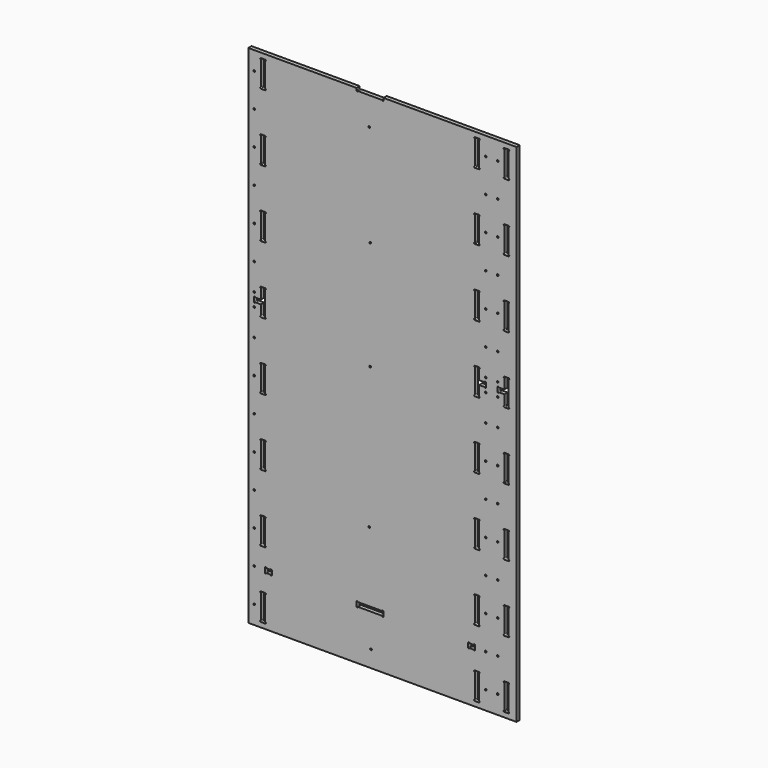
from build123d import *

# Parameters (mm, degrees)
F1_DEPTH = 18


# Not quite as in the source:
# - ends of sketch curves that miss each other by under 0.0002 mm in the source are joined


with BuildPart() as f1:
    # F0 (on Front) → F1 (new body)
    with BuildSketch(Plane.XZ):
        with BuildLine():
            Line((-600, 1063.948714), (-600, -1200))
            Line((-600, -1200), (599.500365, -1200))
            Line((599.500365, -1200), (599.501201, 1063.948476))
            Line((599.501201, 1063.948476), (4.500944, 1063.948707))
            Line((4.500944, 1063.948707), (4.50094, 1053.807502))
            ThreePointArc((4.50094, 1053.807502), (1.3610651837, 1050.5497977616), (-2.0190599785, 1053.5574880017))
            Line((-2.0190599785, 1053.5574880017), (-109.479176, 1053.557255))
            ThreePointArc((-109.479176, 1053.557255), (-112.8596545912, 1050.5399849452), (-115.9991760941, 1053.8072410001))
            Line((-115.9991760941, 1053.8072410001), (-115.999176, 1063.948687))
            Line((-115.999176, 1063.948687), (-600, 1063.948714))
        make_face()
        with BuildLine():
            ThreePointArc((-573.383933, -1114.274894), (-570.7322825706, -1115.3732435706), (-569.633933, -1118.024894))
            ThreePointArc((-569.633933, -1118.024894), (-570.7322825706, -1120.6765444294), (-573.383933, -1121.774894))
            ThreePointArc((-573.383933, -1121.774894), (-576.0355834294, -1120.6765444294), (-577.133933, -1118.024894))
            ThreePointArc((-577.133933, -1118.024894), (-576.0355834294, -1115.3732435706), (-573.383933, -1114.274894))
        make_face(mode=Mode.SUBTRACT)
        with BuildLine():
            ThreePointArc((-543.7502670069, -1064.0442210894), (-546.7588704515, -1060.6682126778), (-543.500265, -1057.5328310434))
            Line((-543.500265, -1057.5328310434), (-525.000247, -1057.532838))
            ThreePointArc((-525.000247, -1057.532838), (-521.7426305, -1060.6682591922), (-524.7502490411, -1064.0442274664))
            Line((-524.7502490411, -1064.0442274664), (-524.750289, -1172.021568))
            ThreePointArc((-524.750289, -1172.021568), (-521.7416865676, -1175.3975768203), (-525.000292, -1178.5329579566))
            Line((-525.000292, -1178.5329579566), (-543.50031, -1178.532951))
            ThreePointArc((-543.50031, -1178.532951), (-546.7579265191, -1175.3975293096), (-543.7503069648, -1172.021561457))
            Line((-543.7503069648, -1172.021561457), (-543.7502670069, -1064.0442210894))
        make_face(mode=Mode.SUBTRACT)
        with BuildLine():
            ThreePointArc((-573.383933, -964.274894), (-570.7322825706, -965.3732435706), (-569.633933, -968.024894))
            ThreePointArc((-569.633933, -968.024894), (-570.7322825706, -970.6765444294), (-573.383933, -971.774894))
            ThreePointArc((-573.383933, -971.774894), (-576.0355834294, -970.6765444294), (-577.133933, -968.024894))
            ThreePointArc((-577.133933, -968.024894), (-576.0355834294, -965.3732435706), (-573.383933, -964.274894))
        make_face(mode=Mode.SUBTRACT)
        with BuildLine():
            ThreePointArc((-525.7517729621, -958.780464), (-522.6163503118, -955.5228484425), (-519.2403833804, -958.5304690293))
            Line((-519.2403833804, -958.5304690293), (-501.263133, -958.530483))
            ThreePointArc((-501.263133, -958.530483), (-497.8871231819, -955.5218816059), (-494.7517430436, -958.780488))
            Line((-494.7517430436, -958.780488), (-494.751749, -977.284406))
            ThreePointArc((-494.751749, -977.284406), (-497.8871691944, -980.5420234617), (-501.2631383898, -977.534405953))
            Line((-501.2631383898, -977.534405953), (-519.240389, -977.534407))
            ThreePointArc((-519.240389, -977.534407), (-522.6163963244, -980.5430114898), (-525.7517789568, -977.284407))
            Line((-525.7517789568, -977.284407), (-525.7517729621, -958.780464))
        make_face(mode=Mode.SUBTRACT)
        with BuildLine():
            ThreePointArc((-573.383933, -814.274894), (-570.7322825706, -815.3732435706), (-569.633933, -818.024894))
            ThreePointArc((-569.633933, -818.024894), (-570.7322825706, -820.6765444294), (-573.383933, -821.774894))
            ThreePointArc((-573.383933, -821.774894), (-576.0355834294, -820.6765444294), (-577.133933, -818.024894))
            ThreePointArc((-577.133933, -818.024894), (-576.0355834294, -815.3732435706), (-573.383933, -814.274894))
        make_face(mode=Mode.SUBTRACT)
        with BuildLine():
            ThreePointArc((-525.000135, -757.5321180377), (-521.7425184809, -760.6675396904), (-524.7501380352, -764.043507543))
            Line((-524.7501380352, -764.043507543), (-524.750179, -872.020644))
            ThreePointArc((-524.750179, -872.020644), (-521.7415765477, -875.3966522839), (-525.000181, -878.5320329566))
            Line((-525.000181, -878.5320329566), (-543.500198, -878.532027))
            ThreePointArc((-543.500198, -878.532027), (-546.7578145191, -875.3966053096), (-543.7501949648, -872.020637457))
            Line((-543.7501949648, -872.020637457), (-543.750156, -764.043501))
            ThreePointArc((-543.750156, -764.043501), (-546.7587584324, -760.6674921797), (-543.500153, -757.5321110434))
            Line((-543.500153, -757.5321110434), (-525.000135, -757.5321180377))
        make_face(mode=Mode.SUBTRACT)
        with BuildLine():
            ThreePointArc((-573.383933, -664.274894), (-570.7322825706, -665.3732435706), (-569.633933, -668.024894))
            ThreePointArc((-569.633933, -668.024894), (-570.7322825706, -670.6765444294), (-573.383933, -671.774894))
            ThreePointArc((-573.383933, -671.774894), (-576.0355834294, -670.6765444294), (-577.133933, -668.024894))
            ThreePointArc((-577.133933, -668.024894), (-576.0355834294, -665.3732435706), (-573.383933, -664.274894))
        make_face(mode=Mode.SUBTRACT)
        with BuildLine():
            ThreePointArc((-54.784835, -1125.619), (-53.6864854294, -1122.9673495706), (-51.034835, -1121.869))
            ThreePointArc((-51.034835, -1121.869), (-48.3831845706, -1122.9673495706), (-47.284835, -1125.619))
            ThreePointArc((-47.284835, -1125.619), (-48.3831845706, -1128.2706504294), (-51.034835, -1129.369))
            ThreePointArc((-51.034835, -1129.369), (-53.6864854294, -1128.2706504294), (-54.784835, -1125.619))
        make_face(mode=Mode.SUBTRACT)
        with BuildLine():
            ThreePointArc((-109.7399839106, -977.5343350069), (-113.1159923222, -980.5429384515), (-116.2513739566, -977.284333))
            Line((-116.2513739566, -977.284333), (-116.251368, -958.78084))
            ThreePointArc((-116.251368, -958.78084), (-113.1159463096, -955.5232234809), (-109.739978457, -958.5308430352))
            Line((-109.739978457, -958.5308430352), (-1.762634, -958.530882))
            ThreePointArc((-1.762634, -958.530882), (1.6133748203, -955.5222795676), (4.7487559566, -958.780885))
            Line((4.7487559566, -958.780885), (4.74875, -977.284377))
            ThreePointArc((4.74875, -977.284377), (1.6133288078, -980.5419935), (-1.7626394664, -977.5343749589))
            Line((-1.7626394664, -977.5343749589), (-109.7399839106, -977.5343350069))
        make_face(mode=Mode.SUBTRACT)
        with BuildLine():
            ThreePointArc((-62.295835, -646.677873), (-61.1974854294, -644.0262225706), (-58.545835, -642.927873))
            ThreePointArc((-58.545835, -642.927873), (-55.8941845706, -644.0262225706), (-54.795835, -646.677873))
            ThreePointArc((-54.795835, -646.677873), (-55.8941845706, -649.3295234294), (-58.545835, -650.427873))
            ThreePointArc((-58.545835, -650.427873), (-61.1974854294, -649.3295234294), (-62.295835, -646.677873))
        make_face(mode=Mode.SUBTRACT)
        with BuildLine():
            ThreePointArc((-573.383933, -514.274894), (-570.7322825706, -515.3732435706), (-569.633933, -518.024894))
            ThreePointArc((-569.633933, -518.024894), (-570.7322825706, -520.6765444294), (-573.383933, -521.774894))
            ThreePointArc((-573.383933, -521.774894), (-576.0355834294, -520.6765444294), (-577.133933, -518.024894))
            ThreePointArc((-577.133933, -518.024894), (-576.0355834294, -515.3732435706), (-573.383933, -514.274894))
        make_face(mode=Mode.SUBTRACT)
        with BuildLine():
            ThreePointArc((-525.000025, -457.5316080377), (-521.7424085015, -460.6670291538), (-524.7500269645, -464.0429974605))
            Line((-524.7500269645, -464.0429974605), (-524.750068, -572.020134))
            ThreePointArc((-524.750068, -572.020134), (-521.7414655477, -575.3961422839), (-525.00007, -578.5315229566))
            Line((-525.00007, -578.5315229566), (-543.500087, -578.531516))
            ThreePointArc((-543.500087, -578.531516), (-546.7577034985, -575.3960948462), (-543.7500850355, -572.0201265395))
            Line((-543.7500850355, -572.0201265395), (-543.750045, -464.04299))
            ThreePointArc((-543.750045, -464.04299), (-546.7586474523, -460.6669817161), (-543.500043, -457.5316010434))
            Line((-543.500043, -457.5316010434), (-525.000025, -457.5316080377))
        make_face(mode=Mode.SUBTRACT)
        with BuildLine():
            ThreePointArc((-573.383933, -364.274894), (-570.7322825706, -365.3732435706), (-569.633933, -368.024894))
            ThreePointArc((-569.633933, -368.024894), (-570.7322825706, -370.6765444294), (-573.383933, -371.774894))
            ThreePointArc((-573.383933, -371.774894), (-576.0355834294, -370.6765444294), (-577.133933, -368.024894))
            ThreePointArc((-577.133933, -368.024894), (-576.0355834294, -365.3732435706), (-573.383933, -364.274894))
        make_face(mode=Mode.SUBTRACT)
        with BuildLine():
            ThreePointArc((-573.383933, -214.274894), (-570.7322825706, -215.3732435706), (-569.633933, -218.024894))
            ThreePointArc((-569.633933, -218.024894), (-570.7322825706, -220.6765444294), (-573.383933, -221.774894))
            ThreePointArc((-573.383933, -221.774894), (-576.0355834294, -220.6765444294), (-577.133933, -218.024894))
            ThreePointArc((-577.133933, -218.024894), (-576.0355834294, -215.3732435706), (-573.383933, -214.274894))
        make_face(mode=Mode.SUBTRACT)
        with BuildLine():
            ThreePointArc((-524.999914, -157.5310970377), (-521.7422974809, -160.6665186904), (-524.7499170352, -164.042486543))
            Line((-524.7499170352, -164.042486543), (-524.749957, -272.019623))
            ThreePointArc((-524.749957, -272.019623), (-521.7413545676, -275.3956318203), (-524.99996, -278.5310129566))
            Line((-524.99996, -278.5310129566), (-543.499977, -278.531006))
            ThreePointArc((-543.499977, -278.531006), (-546.7575935191, -275.3955843096), (-543.7499739648, -272.019616457))
            Line((-543.7499739648, -272.019616457), (-543.749934, -164.04248))
            ThreePointArc((-543.749934, -164.04248), (-546.7585364523, -160.6664717161), (-543.499932, -157.5310910434))
            Line((-543.499932, -157.5310910434), (-524.999914, -157.5310970377))
        make_face(mode=Mode.SUBTRACT)
        with BuildLine():
            ThreePointArc((-573.383933, -64.274894), (-570.7322825706, -65.3732435706), (-569.633933, -68.024894))
            ThreePointArc((-569.633933, -68.024894), (-570.7322825706, -70.6765444294), (-573.383933, -71.774894))
            ThreePointArc((-573.383933, -71.774894), (-576.0355834294, -70.6765444294), (-577.133933, -68.024894))
            ThreePointArc((-577.133933, -68.024894), (-576.0355834294, -65.3732435706), (-573.383933, -64.274894))
        make_face(mode=Mode.SUBTRACT)
        with BuildLine():
            ThreePointArc((-58.540835, -13.997), (-57.4424854294, -11.3453495706), (-54.790835, -10.247))
            ThreePointArc((-54.790835, -10.247), (-52.1391845706, -11.3453495706), (-51.040835, -13.997))
            ThreePointArc((-51.040835, -13.997), (-52.1391845706, -16.6486504294), (-54.790835, -17.747))
            ThreePointArc((-54.790835, -17.747), (-57.4424854294, -16.6486504294), (-58.540835, -13.997))
        make_face(mode=Mode.SUBTRACT)
        with BuildLine():
            ThreePointArc((413.2504909931, -1064.0491890894), (410.2418875485, -1060.6731806778), (413.500493, -1057.5377990434))
            Line((413.500493, -1057.5377990434), (432.000511, -1057.537806))
            ThreePointArc((432.000511, -1057.537806), (435.2581275, -1060.6732271922), (432.2505089589, -1064.0491954664))
            Line((432.2505089589, -1064.0491954664), (432.250469, -1172.026588))
            ThreePointArc((432.250469, -1172.026588), (435.2590714523, -1175.4025962839), (432.000467, -1178.5379769566))
            Line((432.000467, -1178.5379769566), (413.500449, -1178.53797))
            ThreePointArc((413.500449, -1178.53797), (410.2428325, -1175.4025488078), (413.2504510411, -1172.0265805336))
            Line((413.2504510411, -1172.0265805336), (413.2504909931, -1064.0491890894))
        make_face(mode=Mode.SUBTRACT)
        with BuildLine():
            ThreePointArc((389.7605140923, -977.5343449303), (386.3845067161, -980.5429474523), (383.2491260434, -977.284343))
            Line((383.2491260434, -977.284343), (383.249131, -958.781199))
            ThreePointArc((383.249131, -958.781199), (386.3845521922, -955.5235825), (389.7605204664, -958.5312010411))
            Line((389.7605204664, -958.5312010411), (407.737775, -958.531208))
            ThreePointArc((407.737775, -958.531208), (411.1137833222, -955.5226045485), (414.2491649566, -958.78121))
            Line((414.2491649566, -958.78121), (414.249159, -977.284354))
            ThreePointArc((414.249159, -977.284354), (411.1137378462, -980.5419704985), (407.7377695395, -977.5343520355))
            Line((407.7377695395, -977.5343520355), (389.7605140923, -977.5343449303))
        make_face(mode=Mode.SUBTRACT)
        with BuildLine():
            ThreePointArc((461.992664, -1114.274894), (464.6443144294, -1115.3732435706), (465.742664, -1118.024894))
            ThreePointArc((465.742664, -1118.024894), (464.6443144294, -1120.6765444294), (461.992664, -1121.774894))
            ThreePointArc((461.992664, -1121.774894), (459.3410135706, -1120.6765444294), (458.242664, -1118.024894))
            ThreePointArc((458.242664, -1118.024894), (459.3410135706, -1115.3732435706), (461.992664, -1114.274894))
        make_face(mode=Mode.SUBTRACT)
        with BuildLine():
            ThreePointArc((515.501328, -1114.274894), (518.1529784294, -1115.3732435706), (519.251328, -1118.024894))
            ThreePointArc((519.251328, -1118.024894), (518.1529784294, -1120.6765444294), (515.501328, -1121.774894))
            ThreePointArc((515.501328, -1121.774894), (512.8496775706, -1120.6765444294), (511.751328, -1118.024894))
            ThreePointArc((511.751328, -1118.024894), (512.8496775706, -1115.3732435706), (515.501328, -1114.274894))
        make_face(mode=Mode.SUBTRACT)
        with BuildLine():
            Line((545.250583, -1172.026629), (545.250623, -1064.049237))
            ThreePointArc((545.250623, -1064.049237), (542.2420205477, -1060.6732287161), (545.500625, -1057.5378480434))
            Line((545.500625, -1057.5378480434), (564.000643, -1057.537854))
            ThreePointArc((564.000643, -1057.537854), (567.2582595, -1060.6732751922), (564.2506409589, -1064.0492434664))
            Line((564.2506409589, -1064.0492434664), (564.250601, -1172.026636))
            ThreePointArc((564.250601, -1172.026636), (567.2592044515, -1175.4026443222), (564.000599, -1178.5380259566))
            Line((564.000599, -1178.5380259566), (545.500581, -1178.538019))
            ThreePointArc((545.500581, -1178.538019), (542.2429645, -1175.4025978078), (545.250583, -1172.026629))
        make_face(mode=Mode.SUBTRACT)
        with BuildLine():
            ThreePointArc((461.992664, -964.274894), (464.6443144294, -965.3732435706), (465.742664, -968.024894))
            ThreePointArc((465.742664, -968.024894), (464.6443144294, -970.6765444294), (461.992664, -971.774894))
            ThreePointArc((461.992664, -971.774894), (459.3410135706, -970.6765444294), (458.242664, -968.024894))
            ThreePointArc((458.242664, -968.024894), (459.3410135706, -965.3732435706), (461.992664, -964.274894))
        make_face(mode=Mode.SUBTRACT)
        with BuildLine():
            ThreePointArc((515.501328, -964.274894), (518.1529784294, -965.3732435706), (519.251328, -968.024894))
            ThreePointArc((519.251328, -968.024894), (518.1529784294, -970.6765444294), (515.501328, -971.774894))
            ThreePointArc((515.501328, -971.774894), (512.8496775706, -970.6765444294), (511.751328, -968.024894))
            ThreePointArc((511.751328, -968.024894), (512.8496775706, -965.3732435706), (515.501328, -964.274894))
        make_face(mode=Mode.SUBTRACT)
        with BuildLine():
            ThreePointArc((432.000622, -757.5278040377), (435.2582385, -760.6632251922), (432.2506199589, -764.0391934664))
            Line((432.2506199589, -764.0391934664), (432.25058, -872.016382))
            ThreePointArc((432.25058, -872.016382), (435.2591824324, -875.3923908204), (432.0005769998, -878.5277719566))
            Line((432.0005769998, -878.5277719566), (413.50056, -878.527765))
            ThreePointArc((413.50056, -878.527765), (410.2429434809, -875.3923433096), (413.2505630352, -872.016375457))
            Line((413.2505630352, -872.016375457), (413.250602, -764.039187))
            ThreePointArc((413.250602, -764.039187), (410.2419995477, -760.6631787161), (413.500604, -757.5277980434))
            Line((413.500604, -757.5277980434), (432.000622, -757.5278040377))
        make_face(mode=Mode.SUBTRACT)
        with BuildLine():
            ThreePointArc((461.992664, -814.274894), (464.6443144294, -815.3732435706), (465.742664, -818.024894))
            ThreePointArc((465.742664, -818.024894), (464.6443144294, -820.6765444294), (461.992664, -821.774894))
            ThreePointArc((461.992664, -821.774894), (459.3410135706, -820.6765444294), (458.242664, -818.024894))
            ThreePointArc((458.242664, -818.024894), (459.3410135706, -815.3732435706), (461.992664, -814.274894))
        make_face(mode=Mode.SUBTRACT)
        with BuildLine():
            ThreePointArc((515.501328, -814.274894), (518.1529784294, -815.3732435706), (519.251328, -818.024894))
            ThreePointArc((519.251328, -818.024894), (518.1529784294, -820.6765444294), (515.501328, -821.774894))
            ThreePointArc((515.501328, -821.774894), (512.8496775706, -820.6765444294), (511.751328, -818.024894))
            ThreePointArc((511.751328, -818.024894), (512.8496775706, -815.3732435706), (515.501328, -814.274894))
        make_face(mode=Mode.SUBTRACT)
        with BuildLine():
            ThreePointArc((545.500692, -878.5278129623), (542.2430754809, -875.3923913096), (545.2506950352, -872.016423457))
            Line((545.2506950352, -872.016423457), (545.250735, -764.039236))
            ThreePointArc((545.250735, -764.039236), (542.2421315485, -760.6632276778), (545.500737, -757.5278460434))
            Line((545.500737, -757.5278460434), (564.000755, -757.527853))
            ThreePointArc((564.000755, -757.527853), (567.2583715, -760.6632741922), (564.2507529589, -764.0392424664))
            Line((564.2507529589, -764.0392424664), (564.250713, -872.01643))
            ThreePointArc((564.250713, -872.01643), (567.2593154324, -875.3924388203), (564.00071, -878.5278199566))
            Line((564.00071, -878.5278199566), (545.500692, -878.5278129623))
        make_face(mode=Mode.SUBTRACT)
        with BuildLine():
            ThreePointArc((461.992664, -664.274894), (464.6443144294, -665.3732435706), (465.742664, -668.024894))
            ThreePointArc((465.742664, -668.024894), (464.6443144294, -670.6765444294), (461.992664, -671.774894))
            ThreePointArc((461.992664, -671.774894), (459.3410135706, -670.6765444294), (458.242664, -668.024894))
            ThreePointArc((458.242664, -668.024894), (459.3410135706, -665.3732435706), (461.992664, -664.274894))
        make_face(mode=Mode.SUBTRACT)
        with BuildLine():
            ThreePointArc((515.501328, -664.274894), (518.1529784294, -665.3732435706), (519.251328, -668.024894))
            ThreePointArc((519.251328, -668.024894), (518.1529784294, -670.6765444294), (515.501328, -671.774894))
            ThreePointArc((515.501328, -671.774894), (512.8496775706, -670.6765444294), (511.751328, -668.024894))
            ThreePointArc((511.751328, -668.024894), (512.8496775706, -665.3732435706), (515.501328, -664.274894))
        make_face(mode=Mode.SUBTRACT)
        with BuildLine():
            ThreePointArc((432.2506899303, -572.0158729077), (435.2592924523, -575.3918802839), (432.000688, -578.5272609566))
            Line((432.000688, -578.5272609566), (413.500671, -578.527254))
            ThreePointArc((413.500671, -578.527254), (410.2430545015, -575.3918328462), (413.2506729645, -572.0158645395))
            Line((413.2506729645, -572.0158645395), (413.250712, -464.038677))
            ThreePointArc((413.250712, -464.038677), (410.2421095676, -460.6626681797), (413.500715, -457.5272870434))
            Line((413.500715, -457.5272870434), (432.000733, -457.527294))
            ThreePointArc((432.000733, -457.527294), (435.2583495191, -460.6627156904), (432.2507299648, -464.038683543))
            Line((432.2507299648, -464.038683543), (432.2506899303, -572.0158729077))
        make_face(mode=Mode.SUBTRACT)
        with BuildLine():
            ThreePointArc((461.992664, -514.274894), (464.6443144294, -515.3732435706), (465.742664, -518.024894))
            ThreePointArc((465.742664, -518.024894), (464.6443144294, -520.6765444294), (461.992664, -521.774894))
            ThreePointArc((461.992664, -521.774894), (459.3410135706, -520.6765444294), (458.242664, -518.024894))
            ThreePointArc((458.242664, -518.024894), (459.3410135706, -515.3732435706), (461.992664, -514.274894))
        make_face(mode=Mode.SUBTRACT)
        with BuildLine():
            ThreePointArc((515.501328, -514.274894), (518.1529784294, -515.3732435706), (519.251328, -518.024894))
            ThreePointArc((519.251328, -518.024894), (518.1529784294, -520.6765444294), (515.501328, -521.774894))
            ThreePointArc((515.501328, -521.774894), (512.8496775706, -520.6765444294), (511.751328, -518.024894))
            ThreePointArc((511.751328, -518.024894), (512.8496775706, -515.3732435706), (515.501328, -514.274894))
        make_face(mode=Mode.SUBTRACT)
        with BuildLine():
            ThreePointArc((545.500802, -578.5275069623), (542.2431855015, -575.3920858462), (545.2508039645, -572.0161175395))
            Line((545.2508039645, -572.0161175395), (545.250844, -464.038726))
            ThreePointArc((545.250844, -464.038726), (542.2422415676, -460.6627171797), (545.500847, -457.5273360434))
            Line((545.500847, -457.5273360434), (564.000865, -457.527343))
            ThreePointArc((564.000865, -457.527343), (567.2584815191, -460.6627646904), (564.2508619648, -464.038732543))
            Line((564.2508619648, -464.038732543), (564.250822, -572.016125))
            ThreePointArc((564.250822, -572.016125), (567.2594244523, -575.3921332839), (564.00082, -578.5275139566))
            Line((564.00082, -578.5275139566), (545.500802, -578.5275069623))
        make_face(mode=Mode.SUBTRACT)
        with BuildLine():
            ThreePointArc((461.992664, -364.274894), (464.6443144294, -365.3732435706), (465.742664, -368.024894))
            ThreePointArc((465.742664, -368.024894), (464.6443144294, -370.6765444294), (461.992664, -371.774894))
            ThreePointArc((461.992664, -371.774894), (459.3410135706, -370.6765444294), (458.242664, -368.024894))
            ThreePointArc((458.242664, -368.024894), (459.3410135706, -365.3732435706), (461.992664, -364.274894))
        make_face(mode=Mode.SUBTRACT)
        with BuildLine():
            ThreePointArc((515.501328, -364.274894), (518.1529784294, -365.3732435706), (519.251328, -368.024894))
            ThreePointArc((519.251328, -368.024894), (518.1529784294, -370.6765444294), (515.501328, -371.774894))
            ThreePointArc((515.501328, -371.774894), (512.8496775706, -370.6765444294), (511.751328, -368.024894))
            ThreePointArc((511.751328, -368.024894), (512.8496775706, -365.3732435706), (515.501328, -364.274894))
        make_face(mode=Mode.SUBTRACT)
        with BuildLine():
            ThreePointArc((432.000843, -157.5267840377), (435.2584595, -160.6622051922), (432.2508409589, -164.0381734664))
            Line((432.2508409589, -164.0381734664), (432.250801, -272.015361))
            ThreePointArc((432.250801, -272.015361), (435.2594044515, -275.3913693222), (432.000799, -278.5267509566))
            Line((432.000799, -278.5267509566), (413.500782, -278.526744))
            ThreePointArc((413.500782, -278.526744), (410.2431655, -275.3913228078), (413.2507840411, -272.0153545336))
            Line((413.2507840411, -272.0153545336), (413.250823, -164.038167))
            ThreePointArc((413.250823, -164.038167), (410.2422195485, -160.6621586778), (413.500825, -157.5267770434))
            Line((413.500825, -157.5267770434), (432.000843, -157.5267840377))
        make_face(mode=Mode.SUBTRACT)
        with BuildLine():
            ThreePointArc((461.992664, -214.274894), (464.6443144294, -215.3732435706), (465.742664, -218.024894))
            ThreePointArc((465.742664, -218.024894), (464.6443144294, -220.6765444294), (461.992664, -221.774894))
            ThreePointArc((461.992664, -221.774894), (459.3410135706, -220.6765444294), (458.242664, -218.024894))
            ThreePointArc((458.242664, -218.024894), (459.3410135706, -215.3732435706), (461.992664, -214.274894))
        make_face(mode=Mode.SUBTRACT)
        with BuildLine():
            ThreePointArc((515.501328, -214.274894), (518.1529784294, -215.3732435706), (519.251328, -218.024894))
            ThreePointArc((519.251328, -218.024894), (518.1529784294, -220.6765444294), (515.501328, -221.774894))
            ThreePointArc((515.501328, -221.774894), (512.8496775706, -220.6765444294), (511.751328, -218.024894))
            ThreePointArc((511.751328, -218.024894), (512.8496775706, -215.3732435706), (515.501328, -214.274894))
        make_face(mode=Mode.SUBTRACT)
        with BuildLine():
            ThreePointArc((564.000975, -157.5268330377), (567.2585915, -160.6622541922), (564.2509729589, -164.0382224664))
            Line((564.2509729589, -164.0382224664), (564.250933, -272.015614))
            ThreePointArc((564.250933, -272.015614), (567.2595364515, -275.3916223222), (564.000931, -278.5270039566))
            Line((564.000931, -278.5270039566), (545.500913, -278.526997))
            ThreePointArc((545.500913, -278.526997), (542.2432965, -275.3915758078), (545.2509150411, -272.0156075336))
            Line((545.2509150411, -272.0156075336), (545.250955, -164.038216))
            ThreePointArc((545.250955, -164.038216), (542.2423515485, -160.6622076778), (545.500957, -157.5268260434))
            Line((545.500957, -157.5268260434), (564.000975, -157.5268330377))
        make_face(mode=Mode.SUBTRACT)
        with BuildLine():
            ThreePointArc((461.992664, -64.274894), (464.6443144294, -65.3732435706), (465.742664, -68.024894))
            ThreePointArc((465.742664, -68.024894), (464.6443144294, -70.6765444294), (461.992664, -71.774894))
            ThreePointArc((461.992664, -71.774894), (459.3410135706, -70.6765444294), (458.242664, -68.024894))
            ThreePointArc((458.242664, -68.024894), (459.3410135706, -65.3732435706), (461.992664, -64.274894))
        make_face(mode=Mode.SUBTRACT)
        with BuildLine():
            ThreePointArc((515.501328, -64.274894), (518.1529784294, -65.3732435706), (519.251328, -68.024894))
            ThreePointArc((519.251328, -68.024894), (518.1529784294, -70.6765444294), (515.501328, -71.774894))
            ThreePointArc((515.501328, -71.774894), (512.8496775706, -70.6765444294), (511.751328, -68.024894))
            ThreePointArc((511.751328, -68.024894), (512.8496775706, -65.3732435706), (515.501328, -64.274894))
        make_face(mode=Mode.SUBTRACT)
        with BuildLine():
            ThreePointArc((-573.383933, 55.725106), (-570.7322825706, 54.6267564294), (-569.633933, 51.975106))
            ThreePointArc((-569.633933, 51.975106), (-570.7322825706, 49.3234555706), (-573.383933, 48.225106))
            ThreePointArc((-573.383933, 48.225106), (-576.0355834294, 49.3234555706), (-577.133933, 51.975106))
            ThreePointArc((-577.133933, 51.975106), (-576.0355834294, 54.6267564294), (-573.383933, 55.725106))
        make_face(mode=Mode.SUBTRACT)
        with BuildLine():
            ThreePointArc((-573.383933, 115.725106), (-570.7322825706, 114.6267564294), (-569.633933, 111.975106))
            ThreePointArc((-569.633933, 111.975106), (-570.7322825706, 109.3234555706), (-573.383933, 108.225106))
            ThreePointArc((-573.383933, 108.225106), (-576.0355834294, 109.3234555706), (-577.133933, 111.975106))
            ThreePointArc((-577.133933, 111.975106), (-576.0355834294, 114.6267564294), (-573.383933, 115.725106))
        make_face(mode=Mode.SUBTRACT)
        with BuildLine():
            ThreePointArc((-524.999803, 142.4694129623), (-521.7421864809, 139.3339913096), (-524.7498060352, 135.958023457))
            Line((-524.7498060352, 135.958023457), (-524.749847, 27.980887))
            ThreePointArc((-524.749847, 27.980887), (-521.7412435485, 24.6048786778), (-524.999849, 21.4694970434))
            Line((-524.999849, 21.4694970434), (-543.499866, 21.469504))
            ThreePointArc((-543.499866, 21.469504), (-546.7574825, 24.6049251922), (-543.7498639589, 27.9808934664))
            Line((-543.7498639589, 27.9808934664), (-543.749847, 72.46956))
            Line((-543.749847, 72.46956), (-568.238488, 72.469401))
            ThreePointArc((-568.238488, 72.469401), (-571.6144758305, 69.4607757234), (-574.7498789601, 72.71936))
            Line((-574.7498789601, 72.71936), (-574.749872, 91.21938))
            ThreePointArc((-574.749872, 91.21938), (-571.6144508462, 94.4769964985), (-568.2384825395, 91.4693780355))
            Line((-568.2384825395, 91.4693780355), (-543.749841, 91.469369))
            Line((-543.749841, 91.469369), (-543.749825, 135.95803))
            ThreePointArc((-543.749825, 135.95803), (-546.7584284515, 139.3340383222), (-543.499823, 142.4694199566))
            Line((-543.499823, 142.4694199566), (-524.999803, 142.4694129623))
        make_face(mode=Mode.SUBTRACT)
        with BuildLine():
            ThreePointArc((-573.383933, 235.725106), (-570.7322825706, 234.6267564294), (-569.633933, 231.975106))
            ThreePointArc((-569.633933, 231.975106), (-570.7322825706, 229.3234555706), (-573.383933, 228.225106))
            ThreePointArc((-573.383933, 228.225106), (-576.0355834294, 229.3234555706), (-577.133933, 231.975106))
            ThreePointArc((-577.133933, 231.975106), (-576.0355834294, 234.6267564294), (-573.383933, 235.725106))
        make_face(mode=Mode.SUBTRACT)
        with BuildLine():
            ThreePointArc((-573.383933, 385.725106), (-570.7322825706, 384.6267564294), (-569.633933, 381.975106))
            ThreePointArc((-569.633933, 381.975106), (-570.7322825706, 379.3234555706), (-573.383933, 378.225106))
            ThreePointArc((-573.383933, 378.225106), (-576.0355834294, 379.3234555706), (-577.133933, 381.975106))
            ThreePointArc((-577.133933, 381.975106), (-576.0355834294, 384.6267564294), (-573.383933, 385.725106))
        make_face(mode=Mode.SUBTRACT)
        with BuildLine():
            ThreePointArc((-524.999693, 442.4697639623), (-521.7420765, 439.3343428078), (-524.7496950411, 435.9583745336))
            Line((-524.7496950411, 435.9583745336), (-524.749736, 327.981238))
            ThreePointArc((-524.749736, 327.981238), (-521.7411335676, 324.6052291797), (-524.999739, 321.4698480434))
            Line((-524.999739, 321.4698480434), (-543.499755, 321.469855))
            ThreePointArc((-543.499755, 321.469855), (-546.7573715, 324.6052761922), (-543.7497529589, 327.9812444664))
            Line((-543.7497529589, 327.9812444664), (-543.749713, 435.958381))
            ThreePointArc((-543.749713, 435.958381), (-546.7583164515, 439.3343893222), (-543.499711, 442.4697709566))
            Line((-543.499711, 442.4697709566), (-524.999693, 442.4697639623))
        make_face(mode=Mode.SUBTRACT)
        with BuildLine():
            ThreePointArc((-573.383933, 535.725106), (-570.7322825706, 534.6267564294), (-569.633933, 531.975106))
            ThreePointArc((-569.633933, 531.975106), (-570.7322825706, 529.3234555706), (-573.383933, 528.225106))
            ThreePointArc((-573.383933, 528.225106), (-576.0355834294, 529.3234555706), (-577.133933, 531.975106))
            ThreePointArc((-577.133933, 531.975106), (-576.0355834294, 534.6267564294), (-573.383933, 535.725106))
        make_face(mode=Mode.SUBTRACT)
        Polygon((-119.019569, 112.977778), (-136.576902, 112.977778), (-136.576902, 132.948445), (-119.019569, 132.948445), (-118.525193, 132.945041), (-118.033689, 132.91609), (-117.545989, 132.861984), (-117.063027, 132.783111), (-116.585737, 132.679864), (-116.115053, 132.552632), (-115.651908, 132.401807), (-115.197236, 132.227778), (-114.751969, 132.030937), (-114.317043, 131.811674), (-113.89339, 131.57038), (-113.481944, 131.307445), (-113.083639, 131.02326), (-112.699407, 130.718215), (-112.330184, 130.392702), (-111.976902, 130.047111), (-111.636463, 129.695604), (-111.315392, 129.328674), (-111.014055, 128.947213), (-110.732819, 128.552111), (-110.472052, 128.14426), (-110.232121, 127.724549), (-110.013393, 127.293869), (-109.816236, 126.853111), (-109.641015, 126.403166), (-109.4881, 125.944924), (-109.357857, 125.479275), (-109.250652, 125.007111), (-109.166854, 124.529322), (-109.106829, 124.046799), (-109.070945, 123.560432), (-109.059569, 123.071111), (-109.056599, 122.56955), (-109.079439, 122.070497), (-109.127708, 121.574896), (-109.201027, 121.083695), (-109.299019, 120.597837), (-109.421303, 120.118268), (-109.567502, 119.645933), (-109.737236, 119.181778), (-109.930126, 118.726748), (-110.145793, 118.281788), (-110.383859, 117.847844), (-110.643944, 117.425861), (-110.92567, 117.016784), (-111.228657, 116.621559), (-111.552528, 116.241131), (-111.896902, 115.876445), (-112.25703, 115.532319), (-112.632798, 115.208189), (-113.023285, 114.904427), (-113.427569, 114.621403), (-113.844728, 114.359488), (-114.27384, 114.119054), (-114.713983, 113.900471), (-115.164236, 113.704111), (-115.623676, 113.530345), (-116.091381, 113.379544), (-116.566431, 113.252078), (-117.047902, 113.14832), (-117.534874, 113.068639), (-118.026423, 113.013408), (-118.521629, 112.982997), align=None, mode=Mode.SUBTRACT)
        Polygon((-83.35778, 92.431213), (-83.771569, 92.428445), (-84.191435, 92.425041), (-84.610405, 92.432281), (-85.028287, 92.450088), (-85.444887, 92.478387), (-85.860012, 92.517102), (-86.273469, 92.566158), (-86.685067, 92.625477), (-87.094611, 92.694986), (-87.501908, 92.774608), (-87.906767, 92.864268), (-88.308995, 92.96389), (-88.708397, 93.073398), (-89.104782, 93.192716), (-89.497956, 93.32177), (-89.887727, 93.460482), (-90.273902, 93.608778), (-90.656288, 93.766582), (-91.034692, 93.933818), (-91.408921, 94.11041), (-91.778782, 94.296283), (-92.144083, 94.491361), (-92.504631, 94.695569), (-92.860232, 94.90883), (-93.210694, 95.13107), (-93.555824, 95.362211), (-93.895429, 95.60218), (-94.229316, 95.850899), (-94.557293, 96.108294), (-94.879166, 96.374288), (-95.194743, 96.648806), (-95.50383, 96.931772), (-95.806236, 97.223111), (-96.156096, 97.603393), (-96.495617, 97.991581), (-96.824711, 98.387442), (-97.143288, 98.790742), (-97.451259, 99.201246), (-97.748536, 99.618723), (-98.03503, 100.042936), (-98.310652, 100.473653), (-98.575313, 100.910639), (-98.828924, 101.353661), (-99.071397, 101.802485), (-99.302642, 102.256877), (-99.52257, 102.716603), (-99.731094, 103.181428), (-99.928123, 103.65112), (-100.113569, 104.125445), (-100.287343, 104.604167), (-100.449357, 105.087055), (-100.599521, 105.573873), (-100.737746, 106.064387), (-100.863944, 106.558365), (-100.978026, 107.055572), (-101.079903, 107.555773), (-101.169486, 108.058736), (-101.246686, 108.564227), (-101.311414, 109.07201), (-101.363582, 109.581854), (-101.4031, 110.093523), (-101.42988, 110.606784), (-101.443833, 111.121402), (-101.44487, 111.637145), (-101.432902, 112.153778), (-101.448973, 112.714899), (-101.450751, 113.275089), (-101.438334, 113.834088), (-101.411819, 114.391637), (-101.371304, 114.947478), (-101.316887, 115.50135), (-101.248665, 116.052995), (-101.166736, 116.602153), (-101.071197, 117.148565), (-100.962147, 117.691971), (-100.839683, 118.232113), (-100.703902, 118.768731), (-100.554903, 119.301566), (-100.392782, 119.830358), (-100.217639, 120.354849), (-100.029569, 120.874778), (-99.828671, 121.389887), (-99.615043, 121.899917), (-99.388782, 122.404607), (-99.149986, 122.9037), (-98.898752, 123.396935), (-98.635178, 123.884053), (-98.359362, 124.364796), (-98.071402, 124.838903), (-97.771395, 125.306116), (-97.459439, 125.766174), (-97.135631, 126.21882), (-96.800069, 126.663794), (-96.452851, 127.100835), (-96.094074, 127.529686), (-95.723836, 127.950087), (-95.342236, 128.361778), (-95.056487, 128.652452), (-94.763872, 128.934919), (-94.464585, 129.209099), (-94.158824, 129.474908), (-93.846783, 129.732267), (-93.528659, 129.981092), (-93.204648, 130.221304), (-92.874944, 130.45282), (-92.539744, 130.675558), (-92.199244, 130.889437), (-91.853639, 131.094377), (-91.503126, 131.290294), (-91.1479, 131.477107), (-90.788157, 131.654736), (-90.424092, 131.823098), (-90.055902, 131.982111), (-89.683782, 132.131695), (-89.307929, 132.271768), (-88.928537, 132.402248), (-88.545803, 132.523054), (-88.159923, 132.634104), (-87.771092, 132.735316), (-87.379506, 132.82661), (-86.985361, 132.907903), (-86.588852, 132.979114), (-86.190176, 133.040161), (-85.789529, 133.090964), (-85.387105, 133.131439), (-84.983102, 133.161507), (-84.577714, 133.181085), (-84.171138, 133.190091), (-83.763569, 133.188445), (-83.349321, 133.184771), (-82.936208, 133.170307), (-82.52443, 133.145137), (-82.114183, 133.109346), (-81.705668, 133.063017), (-81.299081, 133.006236), (-80.89462, 132.939086), (-80.492486, 132.861653), (-80.092874, 132.774021), (-79.695984, 132.676273), (-79.302014, 132.568496), (-78.911163, 132.450773), (-78.523627, 132.323188), (-78.139607, 132.185827), (-77.759299, 132.038773), (-77.382902, 131.882111), (-77.010615, 131.715926), (-76.642635, 131.540302), (-76.279161, 131.355323), (-75.920392, 131.161075), (-75.566524, 130.957641), (-75.217758, 130.745105), (-74.87429, 130.523554), (-74.536319, 130.29307), (-74.204043, 130.053738), (-73.877661, 129.805643), (-73.557371, 129.54887), (-73.243371, 129.283502), (-72.935859, 129.009624), (-72.635034, 128.727322), (-72.341093, 128.436678), (-72.054236, 128.137778), (-71.684056, 127.72825), (-71.325077, 127.310335), (-70.977391, 126.884286), (-70.64109, 126.450356), (-70.316265, 126.0088), (-70.003009, 125.55987), (-69.701413, 125.10382), (-69.411569, 124.640903), (-69.133569, 124.171373), (-68.867504, 123.695483), (-68.613466, 123.213487), (-68.371548, 122.725637), (-68.141841, 122.232188), (-67.924436, 121.733393), (-67.719426, 121.229505), (-67.526902, 120.720778), (-67.346957, 120.207465), (-67.179681, 119.689819), (-67.025167, 119.168094), (-66.883506, 118.642544), (-66.754791, 118.113421), (-66.639113, 117.580979), (-66.536564, 117.045472), (-66.447236, 116.507153), (-66.37122, 115.966275), (-66.308608, 115.423092), (-66.259492, 114.877858), (-66.223965, 114.330825), (-66.202117, 113.782247), (-66.19404, 113.232378), (-66.199827, 112.68147), (-66.219569, 112.129778), (-66.21114, 111.61495), (-66.21579, 111.101125), (-66.233429, 110.588539), (-66.263965, 110.077429), (-66.307305, 109.568032), (-66.363358, 109.060585), (-66.432032, 108.555324), (-66.513236, 108.052486), (-66.606876, 107.552309), (-66.712863, 107.055029), (-66.831104, 106.560882), (-66.961506, 106.070106), (-67.103979, 105.582938), (-67.258431, 105.099613), (-67.424769, 104.62037), (-67.602902, 104.145445), (-67.792738, 103.675074), (-67.994186, 103.209495), (-68.207153, 102.748944), (-68.431548, 102.293658), (-68.667279, 101.843874), (-68.914254, 101.399829), (-69.172381, 100.96176), (-69.441569, 100.529903), (-69.721725, 100.104495), (-70.012759, 99.685773), (-70.314578, 99.273975), (-70.62709, 98.869335), (-70.950203, 98.472093), (-71.283827, 98.082483), (-71.627868, 97.700744), (-71.982236, 97.327111), (-72.276142, 97.035898), (-72.576735, 96.75281), (-72.883827, 96.477926), (-73.19723, 96.211325), (-73.516757, 95.953085), (-73.842218, 95.703285), (-74.173426, 95.462004), (-74.510194, 95.22932), (-74.852332, 95.005311), (-75.199654, 94.790057), (-75.551971, 94.583636), (-75.909095, 94.386127), (-76.270838, 94.197608), (-76.637012, 94.018158), (-77.00743, 93.847855), (-77.381902, 93.686778), (-77.760242, 93.535006), (-78.142261, 93.392617), (-78.527771, 93.25969), (-78.916585, 93.136304), (-79.308513, 93.022537), (-79.703369, 92.918467), (-80.100964, 92.824174), (-80.501111, 92.739736), (-80.90362, 92.665232), (-81.308305, 92.60074), (-81.714977, 92.546338), (-82.123449, 92.502106), (-82.533532, 92.468122), (-82.945038, 92.444465), align=None, mode=Mode.SUBTRACT)
        Polygon((-39.112447, 92.431213), (-39.526236, 92.428445), (-39.946102, 92.425041), (-40.365072, 92.432281), (-40.782954, 92.450088), (-41.199553, 92.478387), (-41.614678, 92.517102), (-42.028136, 92.566158), (-42.439733, 92.625477), (-42.849277, 92.694986), (-43.256575, 92.774608), (-43.661434, 92.864268), (-44.063661, 92.96389), (-44.463064, 93.073398), (-44.859449, 93.192716), (-45.252623, 93.32177), (-45.642394, 93.460482), (-46.028569, 93.608778), (-46.410955, 93.766582), (-46.789359, 93.933818), (-47.163588, 94.11041), (-47.533449, 94.296283), (-47.89875, 94.491361), (-48.259297, 94.695569), (-48.614899, 94.90883), (-48.965361, 95.13107), (-49.310491, 95.362211), (-49.650096, 95.60218), (-49.983983, 95.850899), (-50.31196, 96.108294), (-50.633833, 96.374288), (-50.949409, 96.648806), (-51.258497, 96.931772), (-51.560902, 97.223111), (-51.910762, 97.603393), (-52.250284, 97.991581), (-52.579377, 98.387442), (-52.897954, 98.790742), (-53.205926, 99.201246), (-53.503203, 99.618723), (-53.789697, 100.042936), (-54.065319, 100.473653), (-54.32998, 100.910639), (-54.583591, 101.353661), (-54.826064, 101.802485), (-55.057308, 102.256877), (-55.277237, 102.716603), (-55.48576, 103.181428), (-55.682789, 103.65112), (-55.868236, 104.125445), (-56.04201, 104.604167), (-56.204023, 105.087055), (-56.354187, 105.573873), (-56.492413, 106.064387), (-56.618611, 106.558365), (-56.732693, 107.055572), (-56.834569, 107.555773), (-56.924152, 108.058736), (-57.001352, 108.564227), (-57.066081, 109.07201), (-57.118248, 109.581854), (-57.157767, 110.093523), (-57.184547, 110.606784), (-57.1985, 111.121402), (-57.199537, 111.637145), (-57.187569, 112.153778), (-57.20364, 112.714899), (-57.205418, 113.275089), (-57.193001, 113.834088), (-57.166486, 114.391637), (-57.125971, 114.947478), (-57.071553, 115.50135), (-57.003331, 116.052995), (-56.921402, 116.602153), (-56.825864, 117.148565), (-56.716814, 117.691971), (-56.594349, 118.232113), (-56.458569, 118.768731), (-56.30957, 119.301566), (-56.147449, 119.830358), (-55.972305, 120.354849), (-55.784236, 120.874778), (-55.583338, 121.389887), (-55.36971, 121.899917), (-55.143448, 122.404607), (-54.904652, 122.9037), (-54.653418, 123.396935), (-54.389845, 123.884053), (-54.114029, 124.364796), (-53.826069, 124.838903), (-53.526062, 125.306116), (-53.214105, 125.766174), (-52.890297, 126.21882), (-52.554736, 126.663794), (-52.207517, 127.100835), (-51.848741, 127.529686), (-51.478503, 127.950087), (-51.096902, 128.361778), (-50.811154, 128.652452), (-50.518538, 128.934919), (-50.219252, 129.209099), (-49.913491, 129.474908), (-49.60145, 129.732267), (-49.283326, 129.981092), (-48.959314, 130.221304), (-48.629611, 130.45282), (-48.294411, 130.675558), (-47.953911, 130.889437), (-47.608306, 131.094377), (-47.257793, 131.290294), (-46.902567, 131.477107), (-46.542823, 131.654736), (-46.178759, 131.823098), (-45.810569, 131.982111), (-45.438449, 132.131695), (-45.062596, 132.271768), (-44.683204, 132.402248), (-44.30047, 132.523054), (-43.914589, 132.634104), (-43.525758, 132.735316), (-43.134172, 132.82661), (-42.740027, 132.907903), (-42.343519, 132.979114), (-41.944843, 133.040161), (-41.544195, 133.090964), (-41.141772, 133.131439), (-40.737769, 133.161507), (-40.332381, 133.181085), (-39.925804, 133.190091), (-39.518236, 133.188445), (-39.103987, 133.184771), (-38.690875, 133.170307), (-38.279096, 133.145137), (-37.86885, 133.109346), (-37.460334, 133.063017), (-37.053747, 133.006236), (-36.649287, 132.939086), (-36.247152, 132.861653), (-35.847541, 132.774021), (-35.450651, 132.676273), (-35.056681, 132.568496), (-34.665829, 132.450773), (-34.278294, 132.323188), (-33.894273, 132.185827), (-33.513966, 132.038773), (-33.137569, 131.882111), (-32.765282, 131.715926), (-32.397302, 131.540302), (-32.033828, 131.355323), (-31.675058, 131.161075), (-31.321191, 130.957641), (-30.972424, 130.745105), (-30.628956, 130.523554), (-30.290986, 130.29307), (-29.95871, 130.053738), (-29.632328, 129.805643), (-29.312038, 129.54887), (-28.998038, 129.283502), (-28.690526, 129.009624), (-28.3897, 128.727322), (-28.09576, 128.436678), (-27.808902, 128.137778), (-27.438722, 127.72825), (-27.079743, 127.310335), (-26.732057, 126.884286), (-26.395756, 126.450356), (-26.070932, 126.0088), (-25.757676, 125.55987), (-25.45608, 125.10382), (-25.166236, 124.640903), (-24.888235, 124.171373), (-24.62217, 123.695483), (-24.368133, 123.213487), (-24.126215, 122.725637), (-23.896507, 122.232188), (-23.679103, 121.733393), (-23.474093, 121.229505), (-23.281569, 120.720778), (-23.101623, 120.207465), (-22.934348, 119.689819), (-22.779834, 119.168094), (-22.638173, 118.642544), (-22.509458, 118.113421), (-22.39378, 117.580979), (-22.291231, 117.045472), (-22.201902, 116.507153), (-22.125886, 115.966275), (-22.063275, 115.423092), (-22.014159, 114.877858), (-21.978631, 114.330825), (-21.956783, 113.782247), (-21.948707, 113.232378), (-21.954494, 112.68147), (-21.974236, 112.129778), (-21.965806, 111.61495), (-21.970457, 111.101125), (-21.988096, 110.588539), (-22.018631, 110.077429), (-22.061972, 109.568032), (-22.118025, 109.060585), (-22.186699, 108.555324), (-22.267902, 108.052486), (-22.361543, 107.552309), (-22.46753, 107.055029), (-22.58577, 106.560882), (-22.716173, 106.070106), (-22.858646, 105.582938), (-23.013098, 105.099613), (-23.179436, 104.62037), (-23.357569, 104.145445), (-23.547405, 103.675074), (-23.748853, 103.209495), (-23.96182, 102.748944), (-24.186215, 102.293658), (-24.421946, 101.843874), (-24.66892, 101.399829), (-24.927048, 100.96176), (-25.196236, 100.529903), (-25.476392, 100.104495), (-25.767426, 99.685773), (-26.069244, 99.273975), (-26.381756, 98.869335), (-26.70487, 98.472093), (-27.038493, 98.082483), (-27.382535, 97.700744), (-27.736902, 97.327111), (-28.030808, 97.035898), (-28.331402, 96.75281), (-28.638494, 96.477926), (-28.951897, 96.211325), (-29.271423, 95.953085), (-29.596885, 95.703285), (-29.928093, 95.462004), (-30.264861, 95.22932), (-30.606999, 95.005311), (-30.954321, 94.790057), (-31.306638, 94.583636), (-31.663762, 94.386127), (-32.025505, 94.197608), (-32.391679, 94.018158), (-32.762096, 93.847855), (-33.136569, 93.686778), (-33.514909, 93.535006), (-33.896928, 93.392617), (-34.282438, 93.25969), (-34.671251, 93.136304), (-35.06318, 93.022537), (-35.458036, 92.918467), (-35.855631, 92.824174), (-36.255777, 92.739736), (-36.658287, 92.665232), (-37.062972, 92.60074), (-37.469644, 92.546338), (-37.878116, 92.502106), (-38.288199, 92.468122), (-38.699705, 92.444465), align=None, mode=Mode.SUBTRACT)
        with BuildLine():
            ThreePointArc((-58.540835, 474.216), (-57.4424854294, 476.8676504294), (-54.790835, 477.966))
            ThreePointArc((-54.790835, 477.966), (-52.1391845706, 476.8676504294), (-51.040835, 474.216))
            ThreePointArc((-51.040835, 474.216), (-52.1391845706, 471.5643495706), (-54.790835, 470.466))
            ThreePointArc((-54.790835, 470.466), (-57.4424854294, 471.5643495706), (-58.540835, 474.216))
        make_face(mode=Mode.SUBTRACT)
        with BuildLine():
            ThreePointArc((-573.383933, 685.725106), (-570.7322825706, 684.6267564294), (-569.633933, 681.975106))
            ThreePointArc((-569.633933, 681.975106), (-570.7322825706, 679.3234555706), (-573.383933, 678.225106))
            ThreePointArc((-573.383933, 678.225106), (-576.0355834294, 679.3234555706), (-577.133933, 681.975106))
            ThreePointArc((-577.133933, 681.975106), (-576.0355834294, 684.6267564294), (-573.383933, 685.725106))
        make_face(mode=Mode.SUBTRACT)
        with BuildLine():
            ThreePointArc((-524.7496259931, 627.9817480894), (-521.7410225485, 624.6057396778), (-524.999628, 621.4703580434))
            Line((-524.999628, 621.4703580434), (-543.499645, 621.470365))
            ThreePointArc((-543.499645, 621.470365), (-546.7572615191, 624.6057866904), (-543.7496419648, 627.981754543))
            Line((-543.7496419648, 627.981754543), (-543.749603, 735.958891))
            ThreePointArc((-543.749603, 735.958891), (-546.7582054324, 739.3348998203), (-543.4996, 742.4702809566))
            Line((-543.4996, 742.4702809566), (-524.999582, 742.470274))
            ThreePointArc((-524.999582, 742.470274), (-521.7419654809, 739.3348523096), (-524.7495850352, 735.958884457))
            Line((-524.7495850352, 735.958884457), (-524.7496259931, 627.9817480894))
        make_face(mode=Mode.SUBTRACT)
        with BuildLine():
            ThreePointArc((-573.383933, 835.725106), (-570.7322825706, 834.6267564294), (-569.633933, 831.975106))
            ThreePointArc((-569.633933, 831.975106), (-570.7322825706, 829.3234555706), (-573.383933, 828.225106))
            ThreePointArc((-573.383933, 828.225106), (-576.0355834294, 829.3234555706), (-577.133933, 831.975106))
            ThreePointArc((-577.133933, 831.975106), (-576.0355834294, 834.6267564294), (-573.383933, 835.725106))
        make_face(mode=Mode.SUBTRACT)
        with BuildLine():
            ThreePointArc((-573.383933, 985.725106), (-570.7322825706, 984.6267564294), (-569.633933, 981.975106))
            ThreePointArc((-569.633933, 981.975106), (-570.7322825706, 979.3234555706), (-573.383933, 978.225106))
            ThreePointArc((-573.383933, 978.225106), (-576.0355834294, 979.3234555706), (-577.133933, 981.975106))
            ThreePointArc((-577.133933, 981.975106), (-576.0355834294, 984.6267564294), (-573.383933, 985.725106))
        make_face(mode=Mode.SUBTRACT)
        with BuildLine():
            ThreePointArc((-524.7495149931, 927.9822580894), (-521.7409115485, 924.6062496778), (-524.999517, 921.4708680434))
            Line((-524.999517, 921.4708680434), (-543.499534, 921.470875))
            ThreePointArc((-543.499534, 921.470875), (-546.7571505, 924.6062961922), (-543.7495319589, 927.9822644664))
            Line((-543.7495319589, 927.9822644664), (-543.749492, 1035.959401))
            ThreePointArc((-543.749492, 1035.959401), (-546.7580954515, 1039.3354093222), (-543.49949, 1042.4707909566))
            Line((-543.49949, 1042.4707909566), (-524.999472, 1042.470784))
            ThreePointArc((-524.999472, 1042.470784), (-521.7418555, 1039.3353628078), (-524.7494740411, 1035.9593945336))
            Line((-524.7494740411, 1035.9593945336), (-524.7495149931, 927.9822580894))
        make_face(mode=Mode.SUBTRACT)
        with BuildLine():
            ThreePointArc((-62.295835, 928.629), (-61.1974854294, 931.2806504294), (-58.545835, 932.379))
            ThreePointArc((-58.545835, 932.379), (-55.8941845706, 931.2806504294), (-54.795835, 928.629))
            ThreePointArc((-54.795835, 928.629), (-55.8941845706, 925.9773495706), (-58.545835, 924.879))
            ThreePointArc((-58.545835, 924.879), (-61.1974854294, 925.9773495706), (-62.295835, 928.629))
        make_face(mode=Mode.SUBTRACT)
        with BuildLine():
            ThreePointArc((432.250912001, 27.9788200131), (435.2595144324, 24.6028111797), (432.000909, 21.4674300434))
            Line((432.000909, 21.4674300434), (413.500892, 21.467437))
            ThreePointArc((413.500892, 21.467437), (410.2432754809, 24.6028586904), (413.2508950352, 27.978826543))
            Line((413.2508950352, 27.978826543), (413.250933, 135.956014))
            ThreePointArc((413.250933, 135.956014), (410.2423305676, 139.3320228203), (413.500936, 142.4674039566))
            Line((413.500936, 142.4674039566), (432.000954, 142.467397))
            ThreePointArc((432.000954, 142.467397), (435.2585705, 139.3319758078), (432.2509519589, 135.9560075336))
            Line((432.2509519589, 135.9560075336), (432.250936, 91.46753))
            Line((432.250936, 91.46753), (456.739578, 91.467353))
            ThreePointArc((456.739578, 91.467353), (460.1156068484, 94.4759325866), (463.2509659529, 91.217306))
            Line((463.2509659529, 91.217306), (463.250959, 72.717291))
            ThreePointArc((463.250959, 72.717291), (460.1155378078, 69.4596745), (456.7395695336, 72.4672930411))
            Line((456.7395695336, 72.4672930411), (432.250928, 72.467302))
            Line((432.250928, 72.467302), (432.250912001, 27.9788200131))
        make_face(mode=Mode.SUBTRACT)
        with BuildLine():
            ThreePointArc((461.992664, 55.725106), (464.6443144294, 54.6267564294), (465.742664, 51.975106))
            ThreePointArc((465.742664, 51.975106), (464.6443144294, 49.3234555706), (461.992664, 48.225106))
            ThreePointArc((461.992664, 48.225106), (459.3410135706, 49.3234555706), (458.242664, 51.975106))
            ThreePointArc((458.242664, 51.975106), (459.3410135706, 54.6267564294), (461.992664, 55.725106))
        make_face(mode=Mode.SUBTRACT)
        with BuildLine():
            ThreePointArc((515.501328, 55.725106), (518.1529784294, 54.6267564294), (519.251328, 51.975106))
            ThreePointArc((519.251328, 51.975106), (518.1529784294, 49.3234555706), (515.501328, 48.225106))
            ThreePointArc((515.501328, 48.225106), (512.8496775706, 49.3234555706), (511.751328, 51.975106))
            ThreePointArc((511.751328, 51.975106), (512.8496775706, 54.6267564294), (515.501328, 55.725106))
        make_face(mode=Mode.SUBTRACT)
        with BuildLine():
            ThreePointArc((461.992664, 115.725106), (464.6443144294, 114.6267564294), (465.742664, 111.975106))
            ThreePointArc((465.742664, 111.975106), (464.6443144294, 109.3234555706), (461.992664, 108.225106))
            ThreePointArc((461.992664, 108.225106), (459.3410135706, 109.3234555706), (458.242664, 111.975106))
            ThreePointArc((458.242664, 111.975106), (459.3410135706, 114.6267564294), (461.992664, 115.725106))
        make_face(mode=Mode.SUBTRACT)
        with BuildLine():
            ThreePointArc((515.501328, 115.725106), (518.1529784294, 114.6267564294), (519.251328, 111.975106))
            ThreePointArc((519.251328, 111.975106), (518.1529784294, 109.3234555706), (515.501328, 108.225106))
            ThreePointArc((515.501328, 108.225106), (512.8496775706, 109.3234555706), (511.751328, 111.975106))
            ThreePointArc((511.751328, 111.975106), (512.8496775706, 114.6267564294), (515.501328, 115.725106))
        make_face(mode=Mode.SUBTRACT)
        with BuildLine():
            ThreePointArc((545.501024, 21.4673880377), (542.2434074809, 24.6028096904), (545.2510270352, 27.978777543))
            Line((545.2510270352, 27.978777543), (545.251043, 72.46747))
            Line((545.251043, 72.46747), (520.762402, 72.467311))
            ThreePointArc((520.762402, 72.467311), (517.3864141695, 69.4586857234), (514.2510110399, 72.71727))
            Line((514.2510110399, 72.71727), (514.251018, 91.21729))
            ThreePointArc((514.251018, 91.21729), (517.3864391922, 94.4749065), (520.7624074664, 91.4672879589))
            Line((520.7624074664, 91.4672879589), (545.251049, 91.467279))
            Line((545.251049, 91.467279), (545.251065, 135.955966))
            ThreePointArc((545.251065, 135.955966), (542.2424625676, 139.3319748204), (545.5010680002, 142.4673559566))
            Line((545.5010680002, 142.4673559566), (564.001087, 142.467349))
            ThreePointArc((564.001087, 142.467349), (567.2587035191, 139.3319273096), (564.2510839648, 135.955959457))
            Line((564.2510839648, 135.955959457), (564.251044, 27.978771))
            ThreePointArc((564.251044, 27.978771), (567.2596464324, 24.6027621797), (564.001041, 21.4673810434))
            Line((564.001041, 21.4673810434), (545.501024, 21.4673880377))
        make_face(mode=Mode.SUBTRACT)
        with BuildLine():
            ThreePointArc((461.992664, 235.725106), (464.6443144294, 234.6267564294), (465.742664, 231.975106))
            ThreePointArc((465.742664, 231.975106), (464.6443144294, 229.3234555706), (461.992664, 228.225106))
            ThreePointArc((461.992664, 228.225106), (459.3410135706, 229.3234555706), (458.242664, 231.975106))
            ThreePointArc((458.242664, 231.975106), (459.3410135706, 234.6267564294), (461.992664, 235.725106))
        make_face(mode=Mode.SUBTRACT)
        with BuildLine():
            ThreePointArc((515.501328, 235.725106), (518.1529784294, 234.6267564294), (519.251328, 231.975106))
            ThreePointArc((519.251328, 231.975106), (518.1529784294, 229.3234555706), (515.501328, 228.225106))
            ThreePointArc((515.501328, 228.225106), (512.8496775706, 229.3234555706), (511.751328, 231.975106))
            ThreePointArc((511.751328, 231.975106), (512.8496775706, 234.6267564294), (515.501328, 235.725106))
        make_face(mode=Mode.SUBTRACT)
        with BuildLine():
            ThreePointArc((432.2510220069, 327.9855000894), (435.2596254515, 324.6094916778), (432.00102, 321.4741100434))
            Line((432.00102, 321.4741100434), (413.501003, 321.474117))
            ThreePointArc((413.501003, 321.474117), (410.2433865, 324.6095381922), (413.2510050411, 327.9855064664))
            Line((413.2510050411, 327.9855064664), (413.251044, 435.962694))
            ThreePointArc((413.251044, 435.962694), (410.2424405485, 439.3387023222), (413.501046, 442.4740839566))
            Line((413.501046, 442.4740839566), (432.001064, 442.474077))
            ThreePointArc((432.001064, 442.474077), (435.2586805, 439.3386558078), (432.2510619589, 435.9626875336))
            Line((432.2510619589, 435.9626875336), (432.2510220069, 327.9855000894))
        make_face(mode=Mode.SUBTRACT)
        with BuildLine():
            ThreePointArc((461.992664, 385.725106), (464.6443144294, 384.6267564294), (465.742664, 381.975106))
            ThreePointArc((465.742664, 381.975106), (464.6443144294, 379.3234555706), (461.992664, 378.225106))
            ThreePointArc((461.992664, 378.225106), (459.3410135706, 379.3234555706), (458.242664, 381.975106))
            ThreePointArc((458.242664, 381.975106), (459.3410135706, 384.6267564294), (461.992664, 385.725106))
        make_face(mode=Mode.SUBTRACT)
        with BuildLine():
            ThreePointArc((515.501328, 385.725106), (518.1529784294, 384.6267564294), (519.251328, 381.975106))
            ThreePointArc((519.251328, 381.975106), (518.1529784294, 379.3234555706), (515.501328, 378.225106))
            ThreePointArc((515.501328, 378.225106), (512.8496775706, 379.3234555706), (511.751328, 381.975106))
            ThreePointArc((511.751328, 381.975106), (512.8496775706, 384.6267564294), (515.501328, 385.725106))
        make_face(mode=Mode.SUBTRACT)
        with BuildLine():
            ThreePointArc((545.501134, 321.4738640377), (542.2435175, 324.6092851922), (545.2511360411, 327.9852534664))
            Line((545.2511360411, 327.9852534664), (545.251176, 435.962646))
            ThreePointArc((545.251176, 435.962646), (542.2425735477, 439.3386542839), (545.501178, 442.4740349566))
            Line((545.501178, 442.4740349566), (564.001196, 442.474028))
            ThreePointArc((564.001196, 442.474028), (567.2588124985, 439.3386068462), (564.2511940355, 435.9626385395))
            Line((564.2511940355, 435.9626385395), (564.251154, 327.985247))
            ThreePointArc((564.251154, 327.985247), (567.2597574515, 324.6092386778), (564.001152, 321.4738570434))
            Line((564.001152, 321.4738570434), (545.501134, 321.4738640377))
        make_face(mode=Mode.SUBTRACT)
        with BuildLine():
            ThreePointArc((461.992664, 535.725106), (464.6443144294, 534.6267564294), (465.742664, 531.975106))
            ThreePointArc((465.742664, 531.975106), (464.6443144294, 529.3234555706), (461.992664, 528.225106))
            ThreePointArc((461.992664, 528.225106), (459.3410135706, 529.3234555706), (458.242664, 531.975106))
            ThreePointArc((458.242664, 531.975106), (459.3410135706, 534.6267564294), (461.992664, 535.725106))
        make_face(mode=Mode.SUBTRACT)
        with BuildLine():
            ThreePointArc((515.501328, 535.725106), (518.1529784294, 534.6267564294), (519.251328, 531.975106))
            ThreePointArc((519.251328, 531.975106), (518.1529784294, 529.3234555706), (515.501328, 528.225106))
            ThreePointArc((515.501328, 528.225106), (512.8496775706, 529.3234555706), (511.751328, 531.975106))
            ThreePointArc((511.751328, 531.975106), (512.8496775706, 534.6267564294), (515.501328, 535.725106))
        make_face(mode=Mode.SUBTRACT)
        with BuildLine():
            ThreePointArc((432.251133001, 627.9860100131), (435.2597354324, 624.6100011797), (432.00113, 621.4746200434))
            Line((432.00113, 621.4746200434), (413.501113, 621.474627))
            ThreePointArc((413.501113, 621.474627), (410.2434964809, 624.6100486904), (413.2511160352, 627.986016543))
            Line((413.2511160352, 627.986016543), (413.251155, 735.963204))
            ThreePointArc((413.251155, 735.963204), (410.2425515485, 739.3392123222), (413.501157, 742.4745939566))
            Line((413.501157, 742.4745939566), (432.001175, 742.474587))
            ThreePointArc((432.001175, 742.474587), (435.2587915, 739.3391658078), (432.2511729589, 735.9631975336))
            Line((432.2511729589, 735.9631975336), (432.251133001, 627.9860100131))
        make_face(mode=Mode.SUBTRACT)
        with BuildLine():
            ThreePointArc((461.992664, 685.725106), (464.6443144294, 684.6267564294), (465.742664, 681.975106))
            ThreePointArc((465.742664, 681.975106), (464.6443144294, 679.3234555706), (461.992664, 678.225106))
            ThreePointArc((461.992664, 678.225106), (459.3410135706, 679.3234555706), (458.242664, 681.975106))
            ThreePointArc((458.242664, 681.975106), (459.3410135706, 684.6267564294), (461.992664, 685.725106))
        make_face(mode=Mode.SUBTRACT)
        with BuildLine():
            ThreePointArc((515.501328, 685.725106), (518.1529784294, 684.6267564294), (519.251328, 681.975106))
            ThreePointArc((519.251328, 681.975106), (518.1529784294, 679.3234555706), (515.501328, 678.225106))
            ThreePointArc((515.501328, 678.225106), (512.8496775706, 679.3234555706), (511.751328, 681.975106))
            ThreePointArc((511.751328, 681.975106), (512.8496775706, 684.6267564294), (515.501328, 685.725106))
        make_face(mode=Mode.SUBTRACT)
        with BuildLine():
            ThreePointArc((545.501244, 621.4743740377), (542.2436274809, 624.6097956904), (545.2512470352, 627.985763543))
            Line((545.2512470352, 627.985763543), (545.251287, 735.963156))
            ThreePointArc((545.251287, 735.963156), (542.2426845477, 739.3391642839), (545.501289, 742.4745449566))
            Line((545.501289, 742.4745449566), (564.001307, 742.474539))
            ThreePointArc((564.001307, 742.474539), (567.2589235, 739.3391178078), (564.2513049589, 735.9631495336))
            Line((564.2513049589, 735.9631495336), (564.251265, 627.985757))
            ThreePointArc((564.251265, 627.985757), (567.2598674324, 624.6097481797), (564.001262, 621.4743670434))
            Line((564.001262, 621.4743670434), (545.501244, 621.4743740377))
        make_face(mode=Mode.SUBTRACT)
        with BuildLine():
            ThreePointArc((461.992664, 835.725106), (464.6443144294, 834.6267564294), (465.742664, 831.975106))
            ThreePointArc((465.742664, 831.975106), (464.6443144294, 829.3234555706), (461.992664, 828.225106))
            ThreePointArc((461.992664, 828.225106), (459.3410135706, 829.3234555706), (458.242664, 831.975106))
            ThreePointArc((458.242664, 831.975106), (459.3410135706, 834.6267564294), (461.992664, 835.725106))
        make_face(mode=Mode.SUBTRACT)
        with BuildLine():
            ThreePointArc((515.501328, 835.725106), (518.1529784294, 834.6267564294), (519.251328, 831.975106))
            ThreePointArc((519.251328, 831.975106), (518.1529784294, 829.3234555706), (515.501328, 828.225106))
            ThreePointArc((515.501328, 828.225106), (512.8496775706, 829.3234555706), (511.751328, 831.975106))
            ThreePointArc((511.751328, 831.975106), (512.8496775706, 834.6267564294), (515.501328, 835.725106))
        make_face(mode=Mode.SUBTRACT)
        with BuildLine():
            ThreePointArc((432.2512429303, 927.9859070923), (435.2598454523, 924.6098997161), (432.001241, 921.4745190434))
            Line((432.001241, 921.4745190434), (413.501223, 921.474525))
            ThreePointArc((413.501223, 921.474525), (410.2436065, 924.6099461922), (413.2512250411, 927.9859144664))
            Line((413.2512250411, 927.9859144664), (413.251265, 1035.963307))
            ThreePointArc((413.251265, 1035.963307), (410.2426625676, 1039.3393158203), (413.501268, 1042.4746969566))
            Line((413.501268, 1042.4746969566), (432.001287, 1042.47469))
            ThreePointArc((432.001287, 1042.47469), (435.2589035191, 1039.3392683096), (432.2512839648, 1035.963300457))
            Line((432.2512839648, 1035.963300457), (432.2512429303, 927.9859070923))
        make_face(mode=Mode.SUBTRACT)
        with BuildLine():
            ThreePointArc((461.992664, 985.725106), (464.6443144294, 984.6267564294), (465.742664, 981.975106))
            ThreePointArc((465.742664, 981.975106), (464.6443144294, 979.3234555706), (461.992664, 978.225106))
            ThreePointArc((461.992664, 978.225106), (459.3410135706, 979.3234555706), (458.242664, 981.975106))
            ThreePointArc((458.242664, 981.975106), (459.3410135706, 984.6267564294), (461.992664, 985.725106))
        make_face(mode=Mode.SUBTRACT)
        with BuildLine():
            ThreePointArc((515.501328, 985.725106), (518.1529784294, 984.6267564294), (519.251328, 981.975106))
            ThreePointArc((519.251328, 981.975106), (518.1529784294, 979.3234555706), (515.501328, 978.225106))
            ThreePointArc((515.501328, 978.225106), (512.8496775706, 979.3234555706), (511.751328, 981.975106))
            ThreePointArc((511.751328, 981.975106), (512.8496775706, 984.6267564294), (515.501328, 985.725106))
        make_face(mode=Mode.SUBTRACT)
        with BuildLine():
            ThreePointArc((545.501356, 921.4746810377), (542.2437395, 924.6101021922), (545.2513580411, 927.9860704664))
            Line((545.2513580411, 927.9860704664), (545.251398, 1035.963258))
            ThreePointArc((545.251398, 1035.963258), (542.2427955676, 1039.3392668203), (545.501401, 1042.4746479566))
            Line((545.501401, 1042.4746479566), (564.001419, 1042.474641))
            ThreePointArc((564.001419, 1042.474641), (567.2590355191, 1039.3392193096), (564.2514159648, 1035.963251457))
            Line((564.2514159648, 1035.963251457), (564.251376, 927.986064))
            ThreePointArc((564.251376, 927.986064), (567.2599794515, 924.6100556778), (564.001374, 921.4746740434))
            Line((564.001374, 921.4746740434), (545.501356, 921.4746810377))
        make_face(mode=Mode.SUBTRACT)
        Polygon((-84.191435, 92.425041), (-83.771569, 92.428445), (-83.35778, 92.431213), (-82.945038, 92.444465), (-82.533532, 92.468122), (-82.123449, 92.502106), (-81.714977, 92.546338), (-81.308305, 92.60074), (-80.90362, 92.665232), (-80.501111, 92.739736), (-80.100964, 92.824174), (-79.703369, 92.918467), (-79.308513, 93.022537), (-78.916585, 93.136304), (-78.527771, 93.25969), (-78.142261, 93.392617), (-77.760242, 93.535006), (-77.381902, 93.686778), (-77.00743, 93.847855), (-76.637012, 94.018158), (-76.270838, 94.197608), (-75.909095, 94.386127), (-75.551971, 94.583636), (-75.199654, 94.790057), (-74.852332, 95.005311), (-74.510194, 95.22932), (-74.173426, 95.462004), (-73.842218, 95.703285), (-73.516757, 95.953085), (-73.19723, 96.211325), (-72.883827, 96.477926), (-72.576735, 96.75281), (-72.276142, 97.035898), (-71.982236, 97.327111), (-71.627868, 97.700744), (-71.283827, 98.082483), (-70.950203, 98.472093), (-70.62709, 98.869335), (-70.314578, 99.273975), (-70.012759, 99.685773), (-69.721725, 100.104495), (-69.441569, 100.529903), (-69.172381, 100.96176), (-68.914254, 101.399829), (-68.667279, 101.843874), (-68.431548, 102.293658), (-68.207153, 102.748944), (-67.994186, 103.209495), (-67.792738, 103.675074), (-67.602902, 104.145445), (-67.424769, 104.62037), (-67.258431, 105.099613), (-67.103979, 105.582938), (-66.961506, 106.070106), (-66.831104, 106.560882), (-66.712863, 107.055029), (-66.606876, 107.552309), (-66.513236, 108.052486), (-66.432032, 108.555324), (-66.363358, 109.060585), (-66.307305, 109.568032), (-66.263965, 110.077429), (-66.233429, 110.588539), (-66.21579, 111.101125), (-66.21114, 111.61495), (-66.219569, 112.129778), (-66.199827, 112.68147), (-66.19404, 113.232378), (-66.202117, 113.782247), (-66.223965, 114.330825), (-66.259492, 114.877858), (-66.308608, 115.423092), (-66.37122, 115.966275), (-66.447236, 116.507153), (-66.536564, 117.045472), (-66.639113, 117.580979), (-66.754791, 118.113421), (-66.883506, 118.642544), (-67.025167, 119.168094), (-67.179681, 119.689819), (-67.346957, 120.207465), (-67.526902, 120.720778), (-67.719426, 121.229505), (-67.924436, 121.733393), (-68.141841, 122.232188), (-68.371548, 122.725637), (-68.613466, 123.213487), (-68.867504, 123.695483), (-69.133569, 124.171373), (-69.411569, 124.640903), (-69.701413, 125.10382), (-70.003009, 125.55987), (-70.316265, 126.0088), (-70.64109, 126.450356), (-70.977391, 126.884286), (-71.325077, 127.310335), (-71.684056, 127.72825), (-72.054236, 128.137778), (-72.341093, 128.436678), (-72.635034, 128.727322), (-72.935859, 129.009624), (-73.243371, 129.283502), (-73.557371, 129.54887), (-73.877661, 129.805643), (-74.204043, 130.053738), (-74.536319, 130.29307), (-74.87429, 130.523554), (-75.217758, 130.745105), (-75.566524, 130.957641), (-75.920392, 131.161075), (-76.279161, 131.355323), (-76.642635, 131.540302), (-77.010615, 131.715926), (-77.382902, 131.882111), (-77.759299, 132.038773), (-78.139607, 132.185827), (-78.523627, 132.323188), (-78.911163, 132.450773), (-79.302014, 132.568496), (-79.695984, 132.676273), (-80.092874, 132.774021), (-80.492486, 132.861653), (-80.89462, 132.939086), (-81.299081, 133.006236), (-81.705668, 133.063017), (-82.114183, 133.109346), (-82.52443, 133.145137), (-82.936208, 133.170307), (-83.349321, 133.184771), (-83.763569, 133.188445), (-84.171138, 133.190091), (-84.577714, 133.181085), (-84.983102, 133.161507), (-85.387105, 133.131439), (-85.789529, 133.090964), (-86.190176, 133.040161), (-86.588852, 132.979114), (-86.985361, 132.907903), (-87.379506, 132.82661), (-87.771092, 132.735316), (-88.159923, 132.634104), (-88.545803, 132.523054), (-88.928537, 132.402248), (-89.307929, 132.271768), (-89.683782, 132.131695), (-90.055902, 131.982111), (-90.424092, 131.823098), (-90.788157, 131.654736), (-91.1479, 131.477107), (-91.503126, 131.290294), (-91.853639, 131.094377), (-92.199244, 130.889437), (-92.539744, 130.675558), (-92.874944, 130.45282), (-93.204648, 130.221304), (-93.528659, 129.981092), (-93.846783, 129.732267), (-94.158824, 129.474908), (-94.464585, 129.209099), (-94.763872, 128.934919), (-95.056487, 128.652452), (-95.342236, 128.361778), (-95.723836, 127.950087), (-96.094074, 127.529686), (-96.452851, 127.100835), (-96.800069, 126.663794), (-97.135631, 126.21882), (-97.459439, 125.766174), (-97.771395, 125.306116), (-98.071402, 124.838903), (-98.359362, 124.364796), (-98.635178, 123.884053), (-98.898752, 123.396935), (-99.149986, 122.9037), (-99.388782, 122.404607), (-99.615043, 121.899917), (-99.828671, 121.389887), (-100.029569, 120.874778), (-100.217639, 120.354849), (-100.392782, 119.830358), (-100.554903, 119.301566), (-100.703902, 118.768731), (-100.839683, 118.232113), (-100.962147, 117.691971), (-101.071197, 117.148565), (-101.166736, 116.602153), (-101.248665, 116.052995), (-101.316887, 115.50135), (-101.371304, 114.947478), (-101.411819, 114.391637), (-101.438334, 113.834088), (-101.450751, 113.275089), (-101.448973, 112.714899), (-101.432902, 112.153778), (-101.44487, 111.637145), (-101.443833, 111.121402), (-101.42988, 110.606784), (-101.4031, 110.093523), (-101.363582, 109.581854), (-101.311414, 109.07201), (-101.246686, 108.564227), (-101.169486, 108.058736), (-101.079903, 107.555773), (-100.978026, 107.055572), (-100.863944, 106.558365), (-100.737746, 106.064387), (-100.599521, 105.573873), (-100.449357, 105.087055), (-100.287343, 104.604167), (-100.113569, 104.125445), (-99.928123, 103.65112), (-99.731094, 103.181428), (-99.52257, 102.716603), (-99.302642, 102.256877), (-99.071397, 101.802485), (-98.828924, 101.353661), (-98.575313, 100.910639), (-98.310652, 100.473653), (-98.03503, 100.042936), (-97.748536, 99.618723), (-97.451259, 99.201246), (-97.143288, 98.790742), (-96.824711, 98.387442), (-96.495617, 97.991581), (-96.156096, 97.603393), (-95.806236, 97.223111), (-95.50383, 96.931772), (-95.194743, 96.648806), (-94.879166, 96.374288), (-94.557293, 96.108294), (-94.229316, 95.850899), (-93.895429, 95.60218), (-93.555824, 95.362211), (-93.210694, 95.13107), (-92.860232, 94.90883), (-92.504631, 94.695569), (-92.144083, 94.491361), (-91.778782, 94.296283), (-91.408921, 94.11041), (-91.034692, 93.933818), (-90.656288, 93.766582), (-90.273902, 93.608778), (-89.887727, 93.460482), (-89.497956, 93.32177), (-89.104782, 93.192716), (-88.708397, 93.073398), (-88.308995, 92.96389), (-87.906767, 92.864268), (-87.501908, 92.774608), (-87.094611, 92.694986), (-86.685067, 92.625477), (-86.273469, 92.566158), (-85.860012, 92.517102), (-85.444887, 92.478387), (-85.028287, 92.450088), (-84.610405, 92.432281), align=None)
        Polygon((-39.946102, 92.425041), (-39.526236, 92.428445), (-39.112447, 92.431213), (-38.699705, 92.444465), (-38.288199, 92.468122), (-37.878116, 92.502106), (-37.469644, 92.546338), (-37.062972, 92.60074), (-36.658287, 92.665232), (-36.255777, 92.739736), (-35.855631, 92.824174), (-35.458036, 92.918467), (-35.06318, 93.022537), (-34.671251, 93.136304), (-34.282438, 93.25969), (-33.896928, 93.392617), (-33.514909, 93.535006), (-33.136569, 93.686778), (-32.762096, 93.847855), (-32.391679, 94.018158), (-32.025505, 94.197608), (-31.663762, 94.386127), (-31.306638, 94.583636), (-30.954321, 94.790057), (-30.606999, 95.005311), (-30.264861, 95.22932), (-29.928093, 95.462004), (-29.596885, 95.703285), (-29.271423, 95.953085), (-28.951897, 96.211325), (-28.638494, 96.477926), (-28.331402, 96.75281), (-28.030808, 97.035898), (-27.736902, 97.327111), (-27.382535, 97.700744), (-27.038493, 98.082483), (-26.70487, 98.472093), (-26.381756, 98.869335), (-26.069244, 99.273975), (-25.767426, 99.685773), (-25.476392, 100.104495), (-25.196236, 100.529903), (-24.927048, 100.96176), (-24.66892, 101.399829), (-24.421946, 101.843874), (-24.186215, 102.293658), (-23.96182, 102.748944), (-23.748853, 103.209495), (-23.547405, 103.675074), (-23.357569, 104.145445), (-23.179436, 104.62037), (-23.013098, 105.099613), (-22.858646, 105.582938), (-22.716173, 106.070106), (-22.58577, 106.560882), (-22.46753, 107.055029), (-22.361543, 107.552309), (-22.267902, 108.052486), (-22.186699, 108.555324), (-22.118025, 109.060585), (-22.061972, 109.568032), (-22.018631, 110.077429), (-21.988096, 110.588539), (-21.970457, 111.101125), (-21.965806, 111.61495), (-21.974236, 112.129778), (-21.954494, 112.68147), (-21.948707, 113.232378), (-21.956783, 113.782247), (-21.978631, 114.330825), (-22.014159, 114.877858), (-22.063275, 115.423092), (-22.125886, 115.966275), (-22.201902, 116.507153), (-22.291231, 117.045472), (-22.39378, 117.580979), (-22.509458, 118.113421), (-22.638173, 118.642544), (-22.779834, 119.168094), (-22.934348, 119.689819), (-23.101623, 120.207465), (-23.281569, 120.720778), (-23.474093, 121.229505), (-23.679103, 121.733393), (-23.896507, 122.232188), (-24.126215, 122.725637), (-24.368133, 123.213487), (-24.62217, 123.695483), (-24.888235, 124.171373), (-25.166236, 124.640903), (-25.45608, 125.10382), (-25.757676, 125.55987), (-26.070932, 126.0088), (-26.395756, 126.450356), (-26.732057, 126.884286), (-27.079743, 127.310335), (-27.438722, 127.72825), (-27.808902, 128.137778), (-28.09576, 128.436678), (-28.3897, 128.727322), (-28.690526, 129.009624), (-28.998038, 129.283502), (-29.312038, 129.54887), (-29.632328, 129.805643), (-29.95871, 130.053738), (-30.290986, 130.29307), (-30.628956, 130.523554), (-30.972424, 130.745105), (-31.321191, 130.957641), (-31.675058, 131.161075), (-32.033828, 131.355323), (-32.397302, 131.540302), (-32.765282, 131.715926), (-33.137569, 131.882111), (-33.513966, 132.038773), (-33.894273, 132.185827), (-34.278294, 132.323188), (-34.665829, 132.450773), (-35.056681, 132.568496), (-35.450651, 132.676273), (-35.847541, 132.774021), (-36.247152, 132.861653), (-36.649287, 132.939086), (-37.053747, 133.006236), (-37.460334, 133.063017), (-37.86885, 133.109346), (-38.279096, 133.145137), (-38.690875, 133.170307), (-39.103987, 133.184771), (-39.518236, 133.188445), (-39.925804, 133.190091), (-40.332381, 133.181085), (-40.737769, 133.161507), (-41.141772, 133.131439), (-41.544195, 133.090964), (-41.944843, 133.040161), (-42.343519, 132.979114), (-42.740027, 132.907903), (-43.134172, 132.82661), (-43.525758, 132.735316), (-43.914589, 132.634104), (-44.30047, 132.523054), (-44.683204, 132.402248), (-45.062596, 132.271768), (-45.438449, 132.131695), (-45.810569, 131.982111), (-46.178759, 131.823098), (-46.542823, 131.654736), (-46.902567, 131.477107), (-47.257793, 131.290294), (-47.608306, 131.094377), (-47.953911, 130.889437), (-48.294411, 130.675558), (-48.629611, 130.45282), (-48.959314, 130.221304), (-49.283326, 129.981092), (-49.60145, 129.732267), (-49.913491, 129.474908), (-50.219252, 129.209099), (-50.518538, 128.934919), (-50.811154, 128.652452), (-51.096902, 128.361778), (-51.478503, 127.950087), (-51.848741, 127.529686), (-52.207517, 127.100835), (-52.554736, 126.663794), (-52.890297, 126.21882), (-53.214105, 125.766174), (-53.526062, 125.306116), (-53.826069, 124.838903), (-54.114029, 124.364796), (-54.389845, 123.884053), (-54.653418, 123.396935), (-54.904652, 122.9037), (-55.143448, 122.404607), (-55.36971, 121.899917), (-55.583338, 121.389887), (-55.784236, 120.874778), (-55.972305, 120.354849), (-56.147449, 119.830358), (-56.30957, 119.301566), (-56.458569, 118.768731), (-56.594349, 118.232113), (-56.716814, 117.691971), (-56.825864, 117.148565), (-56.921402, 116.602153), (-57.003331, 116.052995), (-57.071553, 115.50135), (-57.125971, 114.947478), (-57.166486, 114.391637), (-57.193001, 113.834088), (-57.205418, 113.275089), (-57.20364, 112.714899), (-57.187569, 112.153778), (-57.199537, 111.637145), (-57.1985, 111.121402), (-57.184547, 110.606784), (-57.157767, 110.093523), (-57.118248, 109.581854), (-57.066081, 109.07201), (-57.001352, 108.564227), (-56.924152, 108.058736), (-56.834569, 107.555773), (-56.732693, 107.055572), (-56.618611, 106.558365), (-56.492413, 106.064387), (-56.354187, 105.573873), (-56.204023, 105.087055), (-56.04201, 104.604167), (-55.868236, 104.125445), (-55.682789, 103.65112), (-55.48576, 103.181428), (-55.277237, 102.716603), (-55.057308, 102.256877), (-54.826064, 101.802485), (-54.583591, 101.353661), (-54.32998, 100.910639), (-54.065319, 100.473653), (-53.789697, 100.042936), (-53.503203, 99.618723), (-53.205926, 99.201246), (-52.897954, 98.790742), (-52.579377, 98.387442), (-52.250284, 97.991581), (-51.910762, 97.603393), (-51.560902, 97.223111), (-51.258497, 96.931772), (-50.949409, 96.648806), (-50.633833, 96.374288), (-50.31196, 96.108294), (-49.983983, 95.850899), (-49.650096, 95.60218), (-49.310491, 95.362211), (-48.965361, 95.13107), (-48.614899, 94.90883), (-48.259297, 94.695569), (-47.89875, 94.491361), (-47.533449, 94.296283), (-47.163588, 94.11041), (-46.789359, 93.933818), (-46.410955, 93.766582), (-46.028569, 93.608778), (-45.642394, 93.460482), (-45.252623, 93.32177), (-44.859449, 93.192716), (-44.463064, 93.073398), (-44.063661, 92.96389), (-43.661434, 92.864268), (-43.256575, 92.774608), (-42.849277, 92.694986), (-42.439733, 92.625477), (-42.028136, 92.566158), (-41.614678, 92.517102), (-41.199553, 92.478387), (-40.782954, 92.450088), (-40.365072, 92.432281), align=None)
        Polygon((-136.576902, 132.948445), (-136.576902, 112.977778), (-119.019569, 112.977778), (-118.521629, 112.982997), (-118.026423, 113.013408), (-117.534874, 113.068639), (-117.047902, 113.14832), (-116.566431, 113.252078), (-116.091381, 113.379544), (-115.623676, 113.530345), (-115.164236, 113.704111), (-114.713983, 113.900471), (-114.27384, 114.119054), (-113.844728, 114.359488), (-113.427569, 114.621403), (-113.023285, 114.904427), (-112.632798, 115.208189), (-112.25703, 115.532319), (-111.896902, 115.876445), (-111.552528, 116.241131), (-111.228657, 116.621559), (-110.92567, 117.016784), (-110.643944, 117.425861), (-110.383859, 117.847844), (-110.145793, 118.281788), (-109.930126, 118.726748), (-109.737236, 119.181778), (-109.567502, 119.645933), (-109.421303, 120.118268), (-109.299019, 120.597837), (-109.201027, 121.083695), (-109.127708, 121.574896), (-109.079439, 122.070497), (-109.056599, 122.56955), (-109.059569, 123.071111), (-109.070945, 123.560432), (-109.106829, 124.046799), (-109.166854, 124.529322), (-109.250652, 125.007111), (-109.357857, 125.479275), (-109.4881, 125.944924), (-109.641015, 126.403166), (-109.816236, 126.853111), (-110.013393, 127.293869), (-110.232121, 127.724549), (-110.472052, 128.14426), (-110.732819, 128.552111), (-111.014055, 128.947213), (-111.315392, 129.328674), (-111.636463, 129.695604), (-111.976902, 130.047111), (-112.330184, 130.392702), (-112.699407, 130.718215), (-113.083639, 131.02326), (-113.481944, 131.307445), (-113.89339, 131.57038), (-114.317043, 131.811674), (-114.751969, 132.030937), (-115.197236, 132.227778), (-115.651908, 132.401807), (-116.115053, 132.552632), (-116.585737, 132.679864), (-117.063027, 132.783111), (-117.545989, 132.861984), (-118.033689, 132.91609), (-118.525193, 132.945041), (-119.019569, 132.948445), align=None)
    extrude(amount=F1_DEPTH)


solid = f1.part
